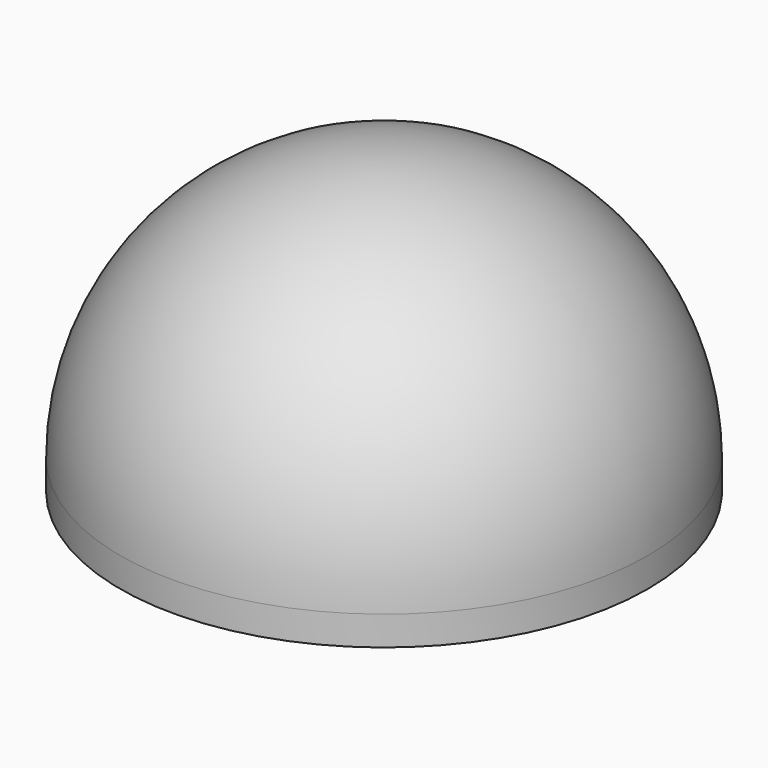
from build123d import *

# Parameters (mm, degrees)
F0_R           = 9
F1_DEPTH       = 1
F3_DEPTH       = 3
F4_R           = 9
F5_DEPTH       = 6
F7_D           = 3.4
F7_DEPTH       = 6
F7_CSINK_D     = 6
F7_CSINK_ANGLE = 100
F7_TIP         = 1.0214630523


# Not quite as in the source:
# - a fillet or chamfer that OpenCascade refuses, or shapes differently, is made with other operations: its cross-section is extruded or revolved along the edge and cut away or added


with BuildPart() as f1:
    # F0 (on Top) → F1 (new body)
    with BuildSketch(Plane.XY):
        Circle(F0_R)
    extrude(amount=F1_DEPTH)

    # F2 (on face) → F3 (join)
    with BuildSketch(Plane.XY.offset(1)):
        with BuildLine():
            Line((2.9, 5.6743157806), (2.9, 1.6743157806))
            Line((2.9, 1.6743157806), (2.9, -1.6743157806))
            Line((2.9, -1.6743157806), (0, -3.3486315613))
            Line((0, -3.3486315613), (-2.9, -1.6743157806))
            Line((-2.9, -1.6743157806), (-2.9, 1.6743157806))
            Line((-2.9, 1.6743157806), (-2.9, 5.6743157806))
            Line((-2.9, 5.6743157806), (-5.2062932022, 7.3412881086))
            ThreePointArc((-5.2062932022, 7.3412881086), (-4.1317890302, -7.995518708), (9, 0))
            ThreePointArc((9, 0), (7.995518708, 4.1317890302), (5.2062932022, 7.3412881086))
            Line((5.2062932022, 7.3412881086), (2.9, 5.6743157806))
        make_face()
    extrude(amount=F3_DEPTH)

    # F4 (on face) → F5 (join)
    with BuildSketch(Plane.XY.offset(4)):
        Circle(F4_R)
    extrude(amount=F5_DEPTH)

    # F6: fillet of radius 9 on 1 edges, made by hand

    # F6_s1 → F6_t2 (revolve, cut)
    with BuildSketch(Plane.XZ):
        with BuildLine():
            ThreePointArc((9, 1), (6.3639610307, 7.3639610307), (0, 10))
            Line((0, 10), (9, 10))
            Line((9, 10), (9, 1))
        make_face()
    revolve(axis=Axis((0, 0, 10), (0, 0, 1)), mode=Mode.SUBTRACT)

    # F7
    with Locations(Plane(origin=(0, 0, 0), x_dir=(1, 0, 0), z_dir=(0, 0, -1))):
        with Locations((0, 0)):
            CounterSinkHole(F7_D / 2, F7_CSINK_D / 2, depth=F7_DEPTH, counter_sink_angle=F7_CSINK_ANGLE)
            with Locations((0, 0, -(F7_DEPTH + F7_TIP / 2))):  # 118° drill point
                Cone(0, F7_D / 2, F7_TIP, mode=Mode.SUBTRACT)


solid = f1.part
